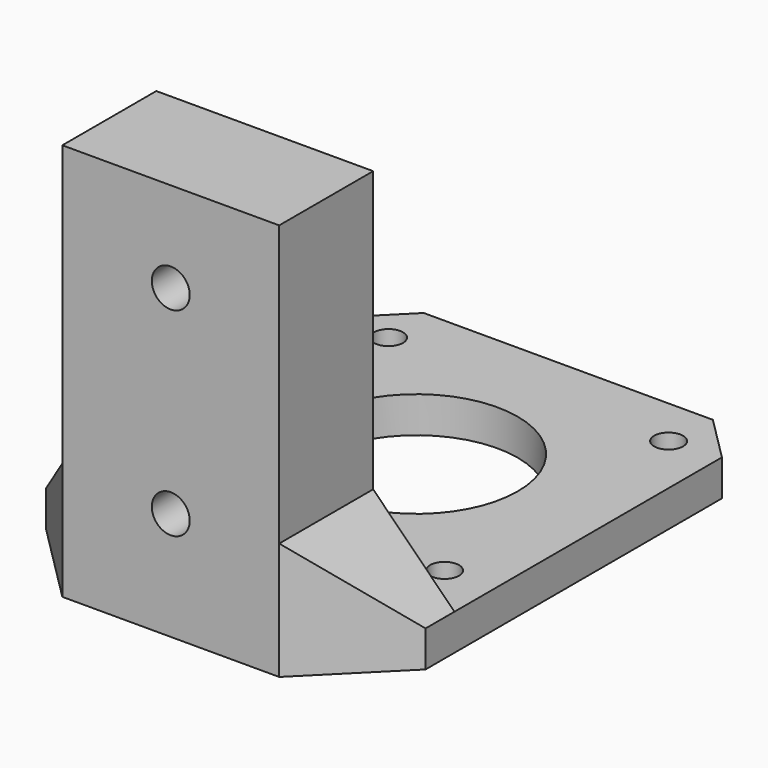
from build123d import *

# Parameters (mm, degrees)
F0_R        = 1.6
F0_R_2      = 11.2
F0_W        = 24
F0_H        = 13
F1_DEPTH    = 4
F2_W        = 24
F2_H        = 13
F3_DEPTH    = 40
F4_T4_DEPTH = 4
F4_T9_DEPTH = 4
F5_SIZE     = 8.99999
F6_R        = 2.1
F7_DEPTH    = 25
F6_R_2      = 4
F8_DEPTH    = 6
F9_SIZE     = 5


# Not quite as in the source:
# - a fillet or chamfer that OpenCascade refuses, or shapes differently, is made with other operations: its cross-section is extruded or revolved along the edge and cut away or added
# - a fillet or chamfer is up to 0.001 mm smaller than in the source, because OpenCascade refuses the exact size


with BuildPart() as f1:
    # F0 (on Top) → F1 (new body)
    with BuildSketch(Plane.XY):
        Polygon((12, -21), (21, -21), (21, 21), (-21, 21), (-21, -21), (-12, -21), align=None)
        with Locations((-15.5, -15.5)):
            Circle(F0_R, mode=Mode.SUBTRACT)
        with Locations((15.5, -15.5)):
            Circle(F0_R, mode=Mode.SUBTRACT)
        with Locations((-15.5, 15.5)):
            Circle(F0_R, mode=Mode.SUBTRACT)
        Circle(F0_R_2, mode=Mode.SUBTRACT)
        with Locations((15.5, 15.5)):
            Circle(F0_R, mode=Mode.SUBTRACT)
        with Locations((0, -27.5)):
            Rectangle(F0_W, F0_H)
    extrude(amount=F1_DEPTH)

    # F2 (on face) → F3 (join)
    with BuildSketch(Plane.XY.offset(4)):
        with Locations((0, -27.5)):
            Rectangle(F2_W, F2_H)
    extrude(amount=F3_DEPTH)

    # F4: chamfer of 13 on 2 edges, made by hand


with BuildPart() as f4_tool2:
    # F4_s3 → F4_t4 (new body)
    with BuildSketch(Plane.XY):
        Polygon((25, -21), (12, -34), (12, -21), align=None)
    extrude(amount=F4_T4_DEPTH)

    split(bisect_by=Plane.YZ.offset(21), keep=Keep.BOTTOM)


with BuildPart() as f1_1:
    add(f1.part)

    # F4_t1: union F4_tool2
    add(f4_tool2.part)


with BuildPart() as f4_tool7:
    # F4_s8 → F4_t9 (new body)
    with BuildSketch(Plane.XY):
        Polygon((-25, -21), (-12, -34), (-12, -21), align=None)
    extrude(amount=F4_T9_DEPTH)

    split(bisect_by=Plane.YZ.offset(-21), keep=Keep.TOP)


with BuildPart() as f1_2:
    add(f1_1.part)

    # F4_t6: union F4_tool7
    add(f4_tool7.part)

    # F5 (size 9 in the source; OpenCascade refuses exactly that, so slightly less here)
    f5_edges = [f1_2.edges().sort_by_distance(p)[0] for p in [
        (12, -27.5, 4),
        (-12, -27.5, 4),
    ]]
    chamfer(f5_edges, length=F5_SIZE)

    # F6 (on face) → F7 (cut)
    with BuildSketch(Plane(origin=(0, -21, 0), x_dir=(-1, 0, 0), z_dir=(0, 1, 0))):
        with Locations((0, 34)):
            Circle(F6_R)
        with Locations((0, 12)):
            Circle(F6_R)
    extrude(amount=-F7_DEPTH, mode=Mode.SUBTRACT)

    # F6 (on face) → F8 (cut)
    with BuildSketch(Plane(origin=(0, -21, 0), x_dir=(-1, 0, 0), z_dir=(0, 1, 0))):
        with Locations((0, 34)):
            Circle(F6_R_2)
        with Locations((0, 34)):
            Circle(F6_R, mode=Mode.SUBTRACT)
        with Locations((0, 12)):
            Circle(F6_R_2)
        with Locations((0, 12)):
            Circle(F6_R, mode=Mode.SUBTRACT)
    extrude(amount=-F8_DEPTH, mode=Mode.SUBTRACT)

    # F9
    f9_edges = [f1_2.edges().sort_by_distance(p)[0] for p in [
        (21, 21, 2),
        (-21, 21, 2),
    ]]
    chamfer(f9_edges, length=F9_SIZE)


solid = f1_2.part
